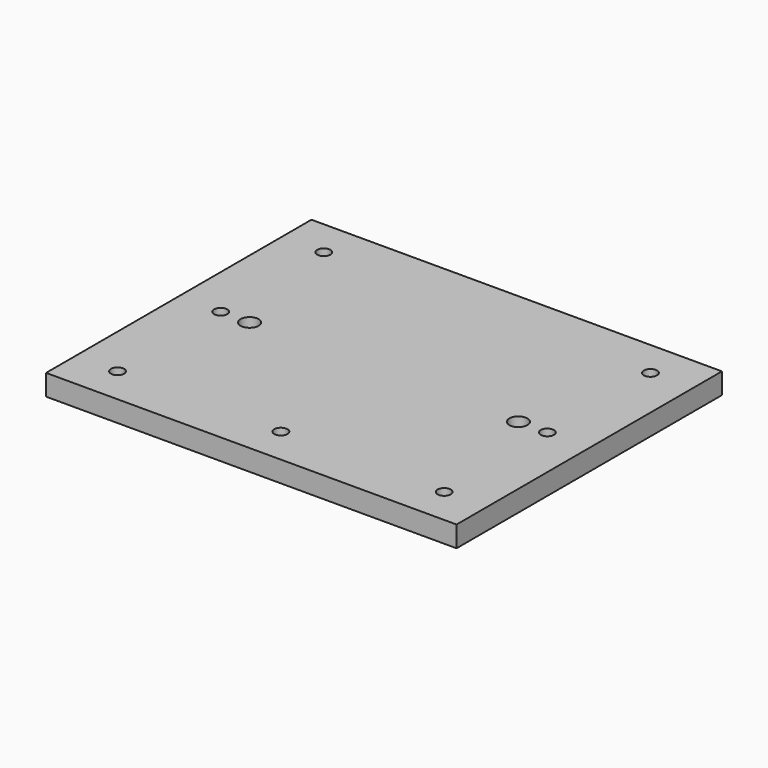
from build123d import *

# Parameters (mm, degrees)
F0_W           = 99.5
F0_H           = 80.4
F1_DEPTH       = 5.08
F3_D           = 4.4
F3_DEPTH       = 38.1
F3_CSINK_D     = 8.96
F3_CSINK_ANGLE = 90
F3_TIP         = 1.3218933619
F5_D           = 3.2
F5_DEPTH       = 37.175
F5_TIP         = 0.9613769904


# Not quite as in the source:
# - a feature names something its author has since deleted; it is built from what else it names


with BuildPart() as f1:
    # F0 (on Top) → F1 (new body)
    with BuildSketch(Plane.XY):
        Rectangle(F0_W, F0_H)
    extrude(amount=F1_DEPTH)

    # F3
    with Locations(Plane(origin=(0, 0, 0), x_dir=(1, 0, 0), z_dir=(0, 0, -1))):
        with Locations((-32.5796, 0), (32.5796, 0)):
            CounterSinkHole(F3_D / 2, F3_CSINK_D / 2, depth=F3_DEPTH, counter_sink_angle=F3_CSINK_ANGLE)
            with Locations((0, 0, -(F3_DEPTH + F3_TIP / 2))):  # 118° drill point
                Cone(0, F3_D / 2, F3_TIP, mode=Mode.SUBTRACT)

    # F5
    with Locations(Plane(origin=(0, 0, 0), x_dir=(1, 0, 0), z_dir=(0, 0, -1))):
        with Locations((-39.59, 31.242), (-39.59, 0), (-39.59, -31.242), (39.59, -31.242), (39.59, 0), (39.59, 31.242), (0, 31.242)):
            Hole(F5_D / 2, depth=F5_DEPTH)
            with Locations((0, 0, -(F5_DEPTH + F5_TIP / 2))):  # 118° drill point
                Cone(0, F5_D / 2, F5_TIP, mode=Mode.SUBTRACT)


solid = f1.part
